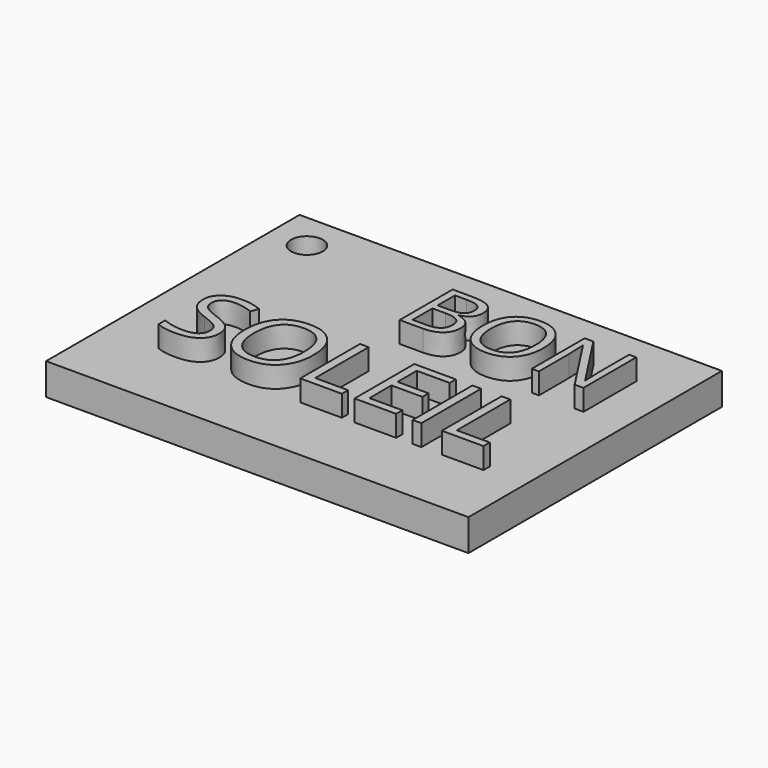
from build123d import *

# Parameters (mm, degrees)
F0_W           = 40
F0_H           = 30
F1_DEPTH       = 3
F2_TEXT_SIZE   = 8.766239302
F2_TEXT_SIZE_2 = 9.9027729852
F3_DEPTH       = 2
F4_R           = 1.5
F5_DEPTH       = 4


# Not quite as in the source:
# - Text() gives the source's letters only with a copy of the font that has no kerning and outlines rounded to 1/6400 em; it was checked with that copy


with BuildPart() as f1:
    # F0 (on Top) → F1 (new body)
    with BuildSketch(Plane.XY):
        with Locations((20, 15)):
            Rectangle(F0_W, F0_H)
    extrude(amount=-F1_DEPTH)

    # F2 (on face) → F3 (join)
    with BuildSketch(Plane.XY):
        with Locations((17.844999209, 18.4802152216)):
            Text('BON', F2_TEXT_SIZE, font='Open Sans', text_align=(TextAlign.LEFT, TextAlign.BOTTOM))
        with Locations((4.6885954216, 6.5807509236)):
            Text('SOLEIL', F2_TEXT_SIZE_2, font='Open Sans', text_align=(TextAlign.LEFT, TextAlign.BOTTOM))
    extrude(amount=F3_DEPTH)

    # F4 (on face) → F5 (cut)
    with BuildSketch(Plane.XY):
        with Locations((3.5, 26.5)):
            Circle(F4_R)
    extrude(amount=-F5_DEPTH, mode=Mode.SUBTRACT)


solid = f1.part
